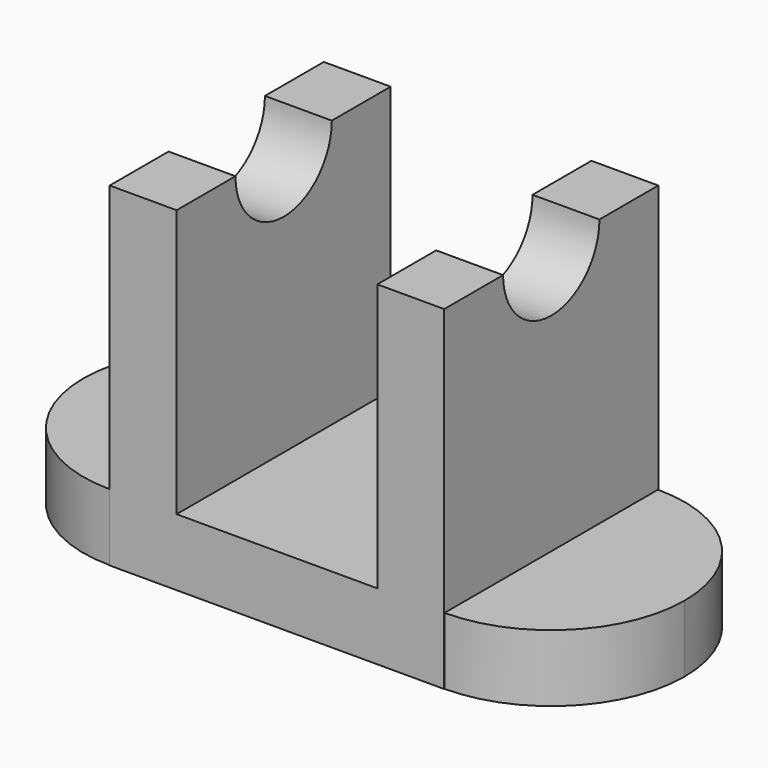
from build123d import *

# Parameters (mm, degrees)
F1_DEPTH = 25.4
F3_DEPTH = 63.501
F5_DEPTH = 12.7


with BuildPart() as f1:
    # F0 (on Front) → F1 (new body, symmetric)
    with BuildSketch(Plane.XZ):
        Polygon((-31.75, 0), (0, 0), (31.75, 0), (31.75, 63.5), (19.05, 63.5), (19.05, 12.7), (0, 12.7), (-19.05, 12.7), (-19.05, 63.5), (-31.75, 63.5), align=None)
    extrude(amount=F1_DEPTH, both=True)

    # F2 (on face) → F3 (cut, through all)
    with BuildSketch(Plane.YZ.offset(31.75)):
        with BuildLine():
            ThreePointArc((-11.43, 63.5), (0, 52.07), (11.43, 63.5))
            Line((11.43, 63.5), (-11.43, 63.5))
        make_face()
    extrude(amount=-F3_DEPTH, mode=Mode.SUBTRACT)

    # F4 (on face) → F5 (join)
    with BuildSketch(Plane(origin=(0, 0, 0), x_dir=(1, 0, 0), z_dir=(0, 0, -1))):
        with BuildLine():
            ThreePointArc((-31.75, -25.3289327497), (-13.8397398924, -17.9102601076), (-6.4210672503, 0))
            ThreePointArc((-6.4210672503, 0), (-13.8397398924, 17.9102601076), (-31.75, 25.3289327497))
            Line((-31.75, 25.3289327497), (-31.75, -25.3289327497))
        make_face()
        with BuildLine():
            Line((-31.75, -25.3289327497), (-31.75, 25.3289327497))
            ThreePointArc((-31.75, 25.3289327497), (-57.0789327497, 0), (-31.75, -25.3289327497))
        make_face()
        with BuildLine():
            ThreePointArc((57.0789327497, 0), (49.6602601076, 17.9102601076), (31.75, 25.3289327497))
            Line((31.75, 25.3289327497), (31.75, -25.3289327497))
            ThreePointArc((31.75, -25.3289327497), (49.6602601076, -17.9102601076), (57.0789327497, 0))
        make_face()
    extrude(amount=-F5_DEPTH)


solid = f1.part
